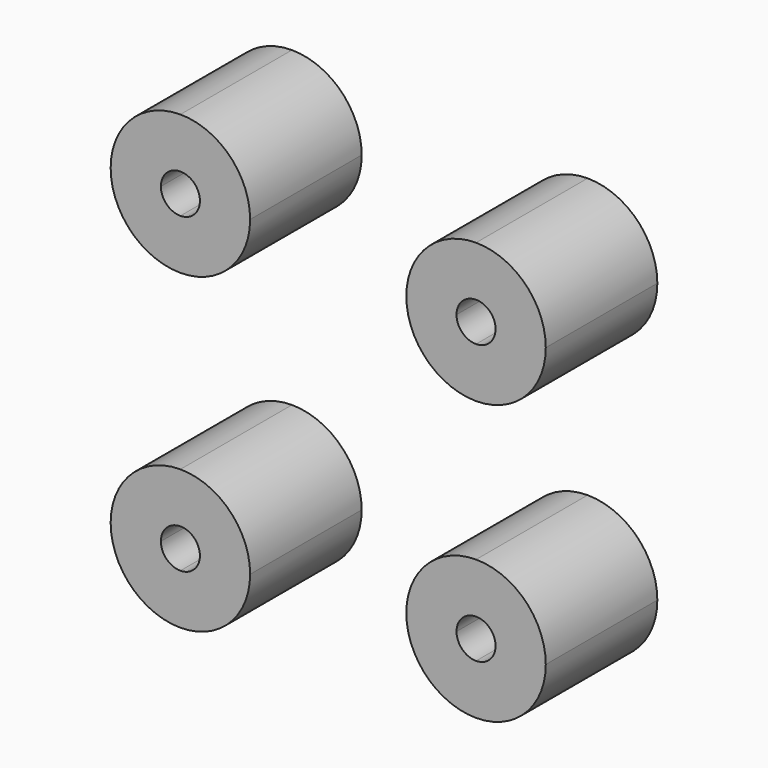
from build123d import *

# Parameters (mm, degrees)
F1_DEPTH = 25.4
F3_DEPTH = 25.4
F5_DEPTH = 25.4
F7_DEPTH = 25.4


# Not quite as in the source:
# - a feature names something its author has since deleted; it is built from what else it names


with BuildPart() as f1:
    # F0 (on Front) → F1 (new body)
    with BuildSketch(Plane.XZ):
        with BuildLine():
            Line((28.956, 25.4), (38.1, 25.4))
            ThreePointArc((38.1, 25.4), (34.3802561211, 34.3802561211), (25.4, 38.1))
            Line((25.4, 38.1), (25.4, 28.956))
            ThreePointArc((25.4, 28.956), (27.9144717139, 27.9144717139), (28.956, 25.4))
        make_face()
        with BuildLine():
            ThreePointArc((25.4, 38.1), (16.4197438789, 34.3802561211), (12.7, 25.4))
            Line((12.7, 25.4), (21.844, 25.4))
            ThreePointArc((21.844, 25.4), (22.8855282861, 27.9144717139), (25.4, 28.956))
            Line((25.4, 28.956), (25.4, 38.1))
        make_face()
        with BuildLine():
            ThreePointArc((12.7, 25.4), (16.4197438789, 16.4197438789), (25.4, 12.7))
            Line((25.4, 12.7), (25.4, 21.844))
            ThreePointArc((25.4, 21.844), (22.8855282861, 22.8855282861), (21.844, 25.4))
            Line((21.844, 25.4), (12.7, 25.4))
        make_face()
        with BuildLine():
            Line((25.4, 21.844), (25.4, 12.7))
            ThreePointArc((25.4, 12.7), (34.3802561211, 16.4197438789), (38.1, 25.4))
            Line((38.1, 25.4), (28.956, 25.4))
            ThreePointArc((28.956, 25.4), (27.9144717139, 22.8855282861), (25.4, 21.844))
        make_face()
    extrude(amount=F1_DEPTH)


with BuildPart() as f3:
    # F2 (on Front) → F3 (new body)
    with BuildSketch(Plane.XZ):
        with BuildLine():
            ThreePointArc((25.4, -38.1), (34.3802561211, -34.3802561211), (38.1, -25.4))
            Line((38.1, -25.4), (28.956, -25.4))
            ThreePointArc((28.956, -25.4), (27.9144717139, -27.9144717139), (25.4, -28.956))
            Line((25.4, -28.956), (25.4, -38.1))
        make_face()
        with BuildLine():
            Line((21.844, -25.4), (12.7, -25.4))
            ThreePointArc((12.7, -25.4), (16.4197438789, -34.3802561211), (25.4, -38.1))
            Line((25.4, -38.1), (25.4, -28.956))
            ThreePointArc((25.4, -28.956), (22.8855282861, -27.9144717139), (21.844, -25.4))
        make_face()
        with BuildLine():
            Line((25.4, -21.844), (25.4, -12.7))
            ThreePointArc((25.4, -12.7), (16.4197438789, -16.4197438789), (12.7, -25.4))
            Line((12.7, -25.4), (21.844, -25.4))
            ThreePointArc((21.844, -25.4), (22.8855282861, -22.8855282861), (25.4, -21.844))
        make_face()
        with BuildLine():
            ThreePointArc((38.1, -25.4), (34.3802561211, -16.4197438789), (25.4, -12.7))
            Line((25.4, -12.7), (25.4, -21.844))
            ThreePointArc((25.4, -21.844), (27.9144717139, -22.8855282861), (28.956, -25.4))
            Line((28.956, -25.4), (38.1, -25.4))
        make_face()
    extrude(amount=F3_DEPTH)


with BuildPart() as f5:
    # F4 (on Front) → F5 (new body)
    with BuildSketch(Plane.XZ):
        with BuildLine():
            ThreePointArc((-28.448, 41.148), (-37.4282561211, 37.4282561211), (-41.148, 28.448))
            Line((-41.148, 28.448), (-32.004, 28.448))
            ThreePointArc((-32.004, 28.448), (-30.9624717139, 30.9624717139), (-28.448, 32.004))
            Line((-28.448, 32.004), (-28.448, 41.148))
        make_face()
        with BuildLine():
            Line((-24.892, 28.448), (-15.748, 28.448))
            ThreePointArc((-15.748, 28.448), (-19.4677438789, 37.4282561211), (-28.448, 41.148))
            Line((-28.448, 41.148), (-28.448, 32.004))
            ThreePointArc((-28.448, 32.004), (-25.9335282861, 30.9624717139), (-24.892, 28.448))
        make_face()
        with BuildLine():
            Line((-28.448, 24.892), (-28.448, 15.748))
            ThreePointArc((-28.448, 15.748), (-19.4677438789, 19.4677438789), (-15.748, 28.448))
            Line((-15.748, 28.448), (-24.892, 28.448))
            ThreePointArc((-24.892, 28.448), (-25.9335282861, 25.9335282861), (-28.448, 24.892))
        make_face()
        with BuildLine():
            ThreePointArc((-41.148, 28.448), (-37.4282561211, 19.4677438789), (-28.448, 15.748))
            Line((-28.448, 15.748), (-28.448, 24.892))
            ThreePointArc((-28.448, 24.892), (-30.9624717139, 25.9335282861), (-32.004, 28.448))
            Line((-32.004, 28.448), (-41.148, 28.448))
        make_face()
    extrude(amount=F5_DEPTH)


with BuildPart() as f7:
    # F6 (on Front) → F7 (new body)
    with BuildSketch(Plane.XZ):
        with BuildLine():
            Line((-28.448, -24.892), (-28.448, -15.748))
            ThreePointArc((-28.448, -15.748), (-37.4282561211, -19.4677438789), (-41.148, -28.448))
            Line((-41.148, -28.448), (-32.004, -28.448))
            ThreePointArc((-32.004, -28.448), (-30.9624717139, -25.9335282861), (-28.448, -24.892))
        make_face()
        with BuildLine():
            Line((-24.892, -28.448), (-15.748, -28.448))
            ThreePointArc((-15.748, -28.448), (-19.4677438789, -19.4677438789), (-28.448, -15.748))
            Line((-28.448, -15.748), (-28.448, -24.892))
            ThreePointArc((-28.448, -24.892), (-25.9335282861, -25.9335282861), (-24.892, -28.448))
        make_face()
        with BuildLine():
            ThreePointArc((-28.448, -41.148), (-19.4677438789, -37.4282561211), (-15.748, -28.448))
            Line((-15.748, -28.448), (-24.892, -28.448))
            ThreePointArc((-24.892, -28.448), (-25.9335282861, -30.9624717139), (-28.448, -32.004))
            Line((-28.448, -32.004), (-28.448, -41.148))
        make_face()
        with BuildLine():
            ThreePointArc((-41.148, -28.448), (-37.4282561211, -37.4282561211), (-28.448, -41.148))
            Line((-28.448, -41.148), (-28.448, -32.004))
            ThreePointArc((-28.448, -32.004), (-30.9624717139, -30.9624717139), (-32.004, -28.448))
            Line((-32.004, -28.448), (-41.148, -28.448))
        make_face()
    extrude(amount=F7_DEPTH)


solid = Compound([f1.part, f3.part, f5.part, f7.part])
